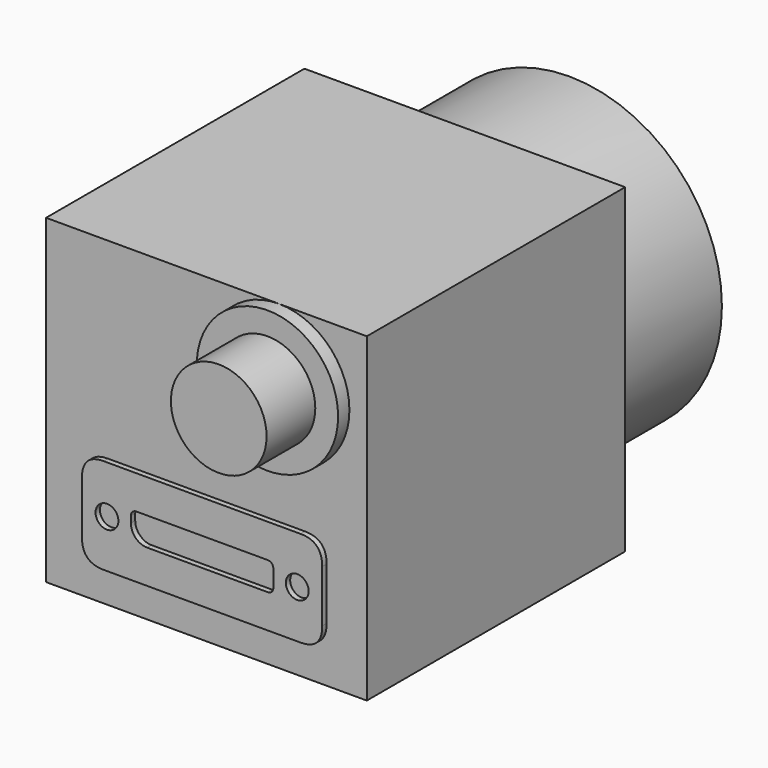
from build123d import *

# Parameters (mm, degrees)
F0_R        = 14.05
F1_DEPTH    = 12
F0_W        = 29.5
F0_H        = 29.5
F2_DEPTH    = 29.7
F3_DEPTH    = 29.7
F5_R        = 6.5
F5_R_2      = 4.4
F6_DEPTH    = 1.3
F7_DEPTH    = 6.9
F5_W        = 22.1
F5_H        = 8.8
F5_W_2      = 13.1
F5_H_2      = 2.6
F8_DEPTH    = 0.5
F9_T1_DEPTH = 5.5
F10_D       = 2.1
F10_DEPTH   = 6.901
F11_R       = 0.5
F12_R       = 1.5


# Not quite as in the source:
# - a fillet or chamfer that OpenCascade refuses, or shapes differently, is made with other operations: its cross-section is extruded or revolved along the edge and cut away or added


with BuildPart() as f1:
    # F0 (on Front) → F1 (new body)
    with BuildSketch(Plane.XZ):
        Circle(F0_R)
    extrude(amount=-F1_DEPTH)

    # F0 (on Front) → F2 (join)
    with BuildSketch(Plane.XZ):
        Rectangle(F0_W, F0_H)
        Circle(F0_R, mode=Mode.SUBTRACT)
    extrude(amount=F2_DEPTH)

    # F0 (on Front) → F3 (join)
    with BuildSketch(Plane.XZ):
        Circle(F0_R)
    extrude(amount=F3_DEPTH)

    # F5 (on offset) → F6 (join)
    with BuildSketch(Plane.XZ.offset(29.7)):
        with Locations((6.65, 8.25)):
            Circle(F5_R)
        with Locations((6.65, 8.25)):
            Circle(F5_R_2, mode=Mode.SUBTRACT)
    extrude(amount=F6_DEPTH)

    # F5 (on offset) → F7 (join)
    with BuildSketch(Plane.XZ.offset(29.7)):
        with Locations((6.65, 8.25)):
            Circle(F5_R_2)
    extrude(amount=F7_DEPTH)

    # F5 (on offset) → F8 (join)
    with BuildSketch(Plane.XZ.offset(29.7)):
        with Locations((6.65, 8.25)):
            Circle(F5_R)
        with Locations((6.65, 8.25)):
            Circle(F5_R_2, mode=Mode.SUBTRACT)
        with Locations((0, -7.3)):
            Rectangle(F5_W, F5_H)
        with Locations((0, -7.3)):
            Rectangle(F5_W_2, F5_H_2, mode=Mode.SUBTRACT)
    extrude(amount=F8_DEPTH)

    # F9: fillet of radius 2 on 4 edges, made by hand

    # F9_s2 → F9_t1 (cut)
    with BuildSketch(Plane.XZ.offset(29.7)):
        with BuildLine():
            add(Edge.make_bspline(
                [(-9.05, -2.9), (-11.05, -2.9), (-11.05, -4.9)],
                knots=[0, 0, 0, 1, 1, 1], degree=2, weights=[1, 1, 1]))
            Line((-11.05, -4.9), (-11.05, -2.9))
            Line((-11.05, -2.9), (-9.05, -2.9))
        make_face()
        with BuildLine():
            add(Edge.make_bspline(
                [(9.05, -2.9), (11.05, -2.9), (11.05, -4.9)],
                knots=[0, 0, 0, 1, 1, 1], degree=2, weights=[1, 1, 1]))
            Line((11.05, -4.9), (11.05, -2.9))
            Line((11.05, -2.9), (9.05, -2.9))
        make_face()
        with BuildLine():
            add(Edge.make_bspline(
                [(-9.05, -11.7), (-11.05, -11.7), (-11.05, -9.7)],
                knots=[0, 0, 0, 1, 1, 1], degree=2, weights=[1, 1, 1]))
            Line((-11.05, -9.7), (-11.05, -11.7))
            Line((-11.05, -11.7), (-9.05, -11.7))
        make_face()
        with BuildLine():
            add(Edge.make_bspline(
                [(11.05, -9.7), (11.05, -11.7), (9.05, -11.7)],
                knots=[0, 0, 0, 1, 1, 1], degree=2, weights=[1, 1, 1]))
            Line((9.05, -11.7), (11.05, -11.7))
            Line((11.05, -11.7), (11.05, -9.7))
        make_face()
    extrude(amount=F9_T1_DEPTH, mode=Mode.SUBTRACT)

    # F10 (through all, one way)
    with BuildSketch(Plane(origin=(0, -29.7, 0), x_dir=(1, 0, 0), z_dir=(0, 1, 0))):
        with Locations((-8.75, 7.3), (8.75, 7.3)):
            Circle(F10_D / 2)
    extrude(amount=-F10_DEPTH, mode=Mode.SUBTRACT)

    # F11
    f11_edges = [f1.edges().sort_by_distance(p)[0] for p in [
        (-6.55, -29.95, -6),
        (6.55, -29.95, -6),
        (6.55, -29.95, -8.6),
    ]]
    fillet(f11_edges, radius=F11_R)

    # F12
    f12_edges = [f1.edges().sort_by_distance(p)[0] for p in [
        (-6.55, -29.95, -8.6),
    ]]
    fillet(f12_edges, radius=F12_R)


solid = f1.part
